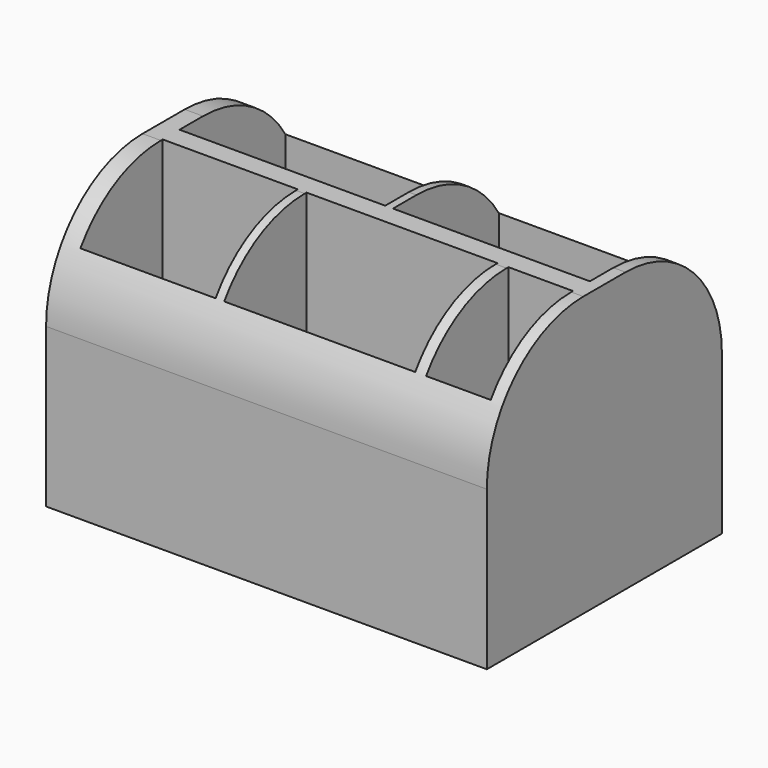
from build123d import *

# Parameters (mm, degrees)
F0_W        = 150
F0_H        = 100
F1_DEPTH    = 95
F2_W        = 70
F2_H        = 45
F2_W_2      = 67
F2_W_3      = 46
F2_H_2      = 35
F2_W_4      = 65
F2_W_5      = 22
F3_DEPTH    = 90
F4_T1_DEPTH = 355.2081528017


# Not quite as in the source:
# - a fillet or chamfer that OpenCascade refuses, or shapes differently, is made with other operations: its cross-section is extruded or revolved along the edge and cut away or added


with BuildPart() as f1:
    # F0 (on Top) → F1 (new body)
    with BuildSketch(Plane.XY):
        with Locations((22.7672072938, 3.643443808)):
            Rectangle(F0_W, F0_H)
    extrude(amount=F1_DEPTH)

    # F2 (on face) → F3 (cut)
    with BuildSketch(Plane.XY.offset(95)):
        with Locations((-11, 25.1181102521)):
            Rectangle(F2_W, F2_H)
        with Locations((60.1440875874, 25.1181102521)):
            Rectangle(F2_W_2, F2_H)
        with Locations((-23, -22.0472425799)):
            Rectangle(F2_W_3, F2_H_2)
        with Locations((35.4433003601, -22.0472425799)):
            Rectangle(F2_W_4, F2_H_2)
        with Locations((82.6440875874, -22.0472425799)):
            Rectangle(F2_W_5, F2_H_2)
    extrude(amount=-F3_DEPTH, mode=Mode.SUBTRACT)

    # F4: fillet of radius 41.0416305603 on 2 edges, made by hand

    # F4_s2 → F4_t1 (cut)
    with BuildSketch(Plane.YZ.offset(-154.8368691071)):
        with BuildLine():
            ThreePointArc((-5.3149256317, 95), (-34.3357409119, 82.9791847198), (-46.356556192, 53.9583694397))
            Line((-46.356556192, 53.9583694397), (-46.356556192, 95))
            Line((-46.356556192, 95), (-5.3149256317, 95))
        make_face()
        with BuildLine():
            ThreePointArc((53.643443808, 53.9583694397), (41.6226285278, 82.9791847198), (12.6018132476, 95))
            Line((12.6018132476, 95), (53.643443808, 95))
            Line((53.643443808, 95), (53.643443808, 53.9583694397))
        make_face()
    extrude(amount=F4_T1_DEPTH, mode=Mode.SUBTRACT)


solid = f1.part
